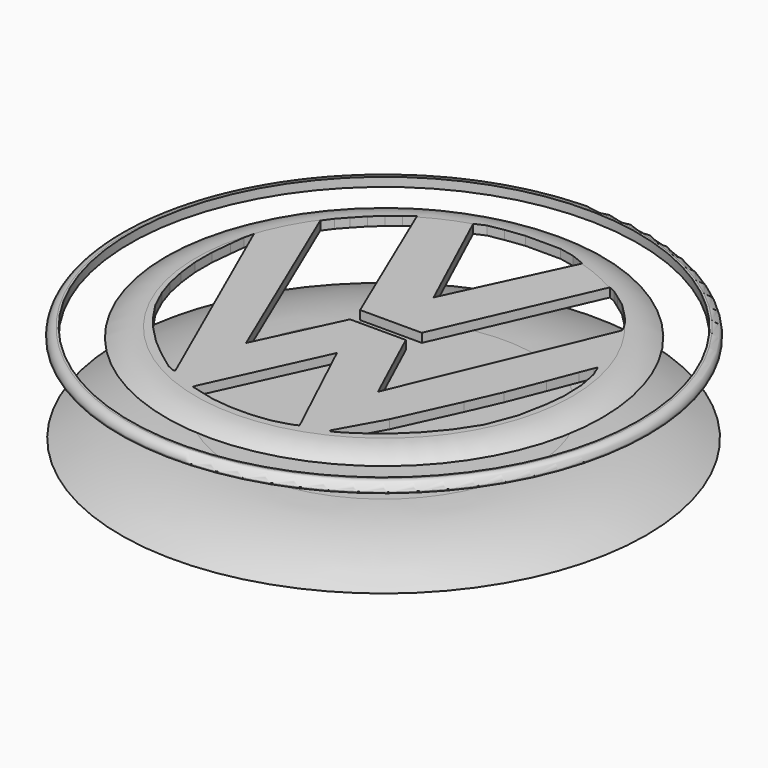
from build123d import *

# Parameters (mm, degrees)
F1_R     = 74.9503094081
F2_DEPTH = 7.112
F5_R     = 75.3033209634
F5_R_2   = 72.5045645267
F6_DEPTH = 2.54
F5_R_3   = 62.2020124847
F7_R     = 2.2075568814


# Not quite as in the source:
# - a fillet or chamfer that OpenCascade refuses, or shapes differently, is made with other operations: its cross-section is extruded or revolved along the edge and cut away or added


with BuildPart() as f2:
    # F1 (on offset) → F2 (new body)
    with BuildSketch(Plane.XY.offset(25.4)):
        with Locations((56.4802102745, 0)):
            Circle(F1_R)
    extrude(amount=F2_DEPTH)

    # F3: fillet of radius 74.93 on 1 edges, made by hand

    # F3_s1 → F3_t2 (revolve, cut)
    with BuildSketch(Plane.XZ):
        with BuildLine():
            ThreePointArc((131.4305196826, 25.4), (115.8912725817, 30.7123891689), (99.5679432645, 32.512))
            Line((99.5679432645, 32.512), (131.4305196826, 32.512))
            Line((131.4305196826, 32.512), (131.4305196826, 25.4))
        make_face()
    revolve(axis=Axis((56.4802102745, 0, 32.512), (0, 0, 1)), mode=Mode.SUBTRACT)


with BuildPart() as f6:
    # F5 (on offset) → F6 (new body)
    with BuildSketch(Plane.XY.offset(50.8)):
        with Locations((56.6154569387, 0)):
            Circle(F5_R)
        with Locations((56.6154569387, 0)):
            Circle(F5_R_2, mode=Mode.SUBTRACT)
    extrude(amount=F6_DEPTH)

    # F7
    f7_edges = [f6.edges().sort_by_distance(p)[0] for p in [
        (-18.687864, 0, 53.34),
    ]]
    fillet(f7_edges, radius=F7_R)


with BuildPart() as f6b:
    # F5 (on offset) → F6, piece 2 (new body)
    with BuildSketch(Plane.XY.offset(50.8)):
        with Locations((56.6154569387, 0)):
            Circle(F5_R_3)
        Polygon((5.2329944447, 14.3430121243), (5.898731295, 16.9798284769), (33.0860838294, -44.6780584753), (33.457006761, -45.4831748782), (33.0860838294, -45.6540617471), (30.8668957569, -44.6780584753), (25.7025100291, -40.8380627632), (21.0224930197, -36.8890799582), (16.4521634579, -32.1722403169), (13.3880926296, -28.332946822), (10.1506058127, -23.4965197742), (7.5493352948, -17.850264491), (5.9764734469, -13.0171226338), (4.8623140901, -7.6890783384), (4.1666254401, -1.8188767135), (4.1666254401, 4.1910852306), (4.7489954159, 10.0860549137), align=None, mode=Mode.SUBTRACT)
        Polygon((41.3734834984, -49.098044961), (41.4462983608, -48.5069826245), (56.2054026438, -16.2932312143), (71.5567991138, -48.7970970571), (70.0133701047, -49.5260500609), (65.2788728476, -50.8655197918), (59.8435918396, -51.5096651804), (54.1100800037, -51.5096651804), (48.4588332474, -50.8869364858), (44.9598932599, -50.0035327991), align=None, mode=Mode.SUBTRACT)
        Polygon((78.4665318757, -46.5765341646), (78.5067006946, -46.165484935), (85.3073447943, -33.952884376), (93.0711701512, -17.0072801411), (97.07782145, -7.8971541512), (101.1134237051, 2.2634342313), (104.1416749358, 10.0860549137), (105.5729240179, 13.7291774154), (105.9481124429, 14.5822623402), (107.3307628276, 11.3282663451), (108.4373518825, 5.7824077085), (108.6700335145, -0.8365057874), (108.1271097064, -6.29193848), (106.5634787083, -14.5498057827), (103.3893972635, -22.8985361755), (99.3457064033, -29.0296357125), (94.8939084716, -34.3055487947), (90.8683389425, -38.205768913), (87.3253419995, -41.2038601935), (83.3948552608, -44.0376214683), (79.9579694867, -46.1400896311), (78.7448983092, -46.6989602687), align=None, mode=Mode.SUBTRACT)
        Polygon((37.3803153634, -25.189589709), (13.3880926296, 31.2748625875), (15.3208132833, 33.910214901), (17.6687631756, 36.5191921592), (20.3645564616, 39.3890663981), (23.2342723757, 41.9980436563), (26.3648722321, 44.4330908358), (28.9003048092, 46.3744103909), (47.2842479364, 3.1087533801), (64.8886337876, 3.1087533801), (83.9169546962, 46.3744103909), (85.736560865, 45.5741440249), (88.1518572569, 43.8337177038), (91.1508873105, 41.6618846357), (94.0464958549, 38.7661121786), (96.6835692525, 35.9220467508), (98.3382090926, 33.3882421255), (98.9849639466, 31.9844115796), (98.8086760044, 31.2748625875), (75.023278594, -25.189589709), (64.2681494355, -1.8178562168), (48.3422763646, -1.8178562168), align=None, mode=Mode.SUBTRACT)
        Polygon((67.9322704673, 53.2166548073), (71.9324797392, 51.5642985702), (56.2794841826, 18.0824100971), (40.9743338823, 51.3034015894), (43.8373587113, 52.6224177702), (48.2790656388, 53.3905848861), (53.6706522107, 54.0863126516), (58.6274340749, 54.0863126516), (63.6711791158, 54.0863126516), align=None, mode=Mode.SUBTRACT)
    extrude(amount=F6_DEPTH)

    # F8: fillet of radius 15.7595032925 on 1 edges, made by hand

    # F8_s1 → F8_t2 (revolve, cut)
    with BuildSketch(Plane.XZ):
        with BuildLine():
            ThreePointArc((118.8174694234, 50.8), (114.711800609, 52.6916639306), (110.2380360665, 53.34))
            Line((110.2380360665, 53.34), (110.2380360665, 53.6551900658))
            Line((110.2380360665, 53.6551900658), (118.8174694234, 53.6551900658))
            Line((118.8174694234, 53.6551900658), (119.1326594893, 53.34))
            ThreePointArc((119.1326594893, 53.34), (119.1326594893, 52.07), (118.9890580906, 51.0643900658))
            Line((118.9890580906, 51.0643900658), (118.8174694234, 50.8))
        make_face()
    revolve(axis=Axis((56.6154569387, 0, 53.34), (0, 0, 1)), mode=Mode.SUBTRACT)


solid = Compound([f2.part, f6.part, f6b.part])
